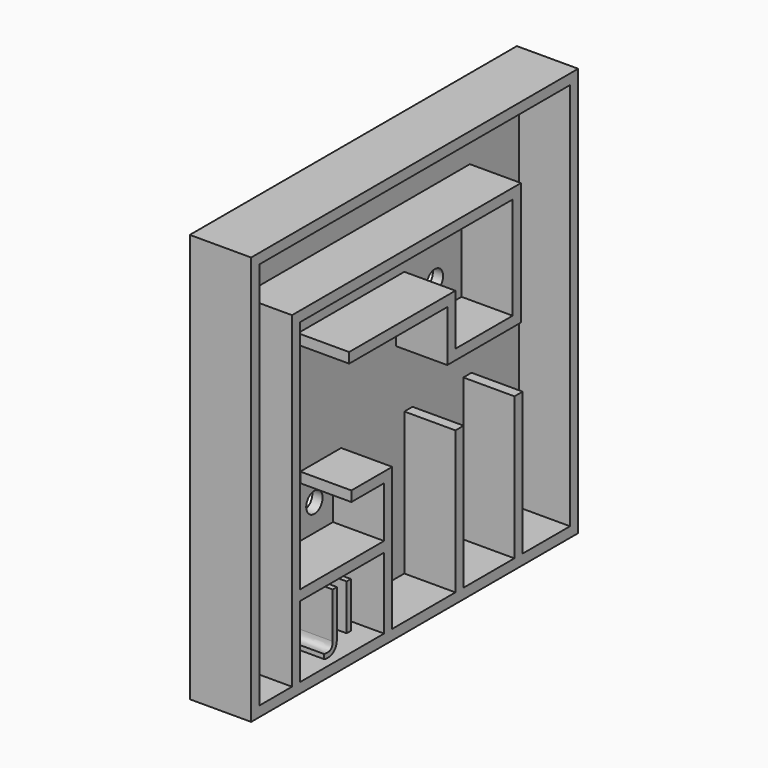
from build123d import *

# Parameters (mm, degrees)
F0_W          = 50.8
F0_H          = 50.8
F1_DEPTH      = 7.62
F2_T          = -1.27
F3_W          = 1.27
F3_H          = 40.64
F4_DEPTH      = 6.35
F5_R          = 1.27
F6_DEPTH      = 2540
F7_DEPTH      = 25.4
F10_DEPTH     = 6.35
F8_W          = 34.29
F8_H          = 1.27
F11_DEPTH     = 6.35
F12_W         = 1.27
F12_H         = 1.27
F12_W_2       = 15.24
F12_W_3       = 5.08
F12_W_4       = 13.0282191968
F12_H_2       = 17.7213940769
F13_DEPTH     = 6.35
F14_TEXT_SIZE = 7.9484365415
F15_DEPTH     = 6.35
F16_R         = 1.27
F17_DEPTH     = 254


# Not quite as in the source:
# - Text() gives the source's letters only with a copy of the font that has no kerning and outlines rounded to 1/6400 em; it was checked with that copy


with BuildPart() as f1:
    # F0 (on Right) → F1 (new body)
    with BuildSketch(Plane.YZ):
        with Locations((-25.4, 25.4)):
            Rectangle(F0_W, F0_H)
    extrude(amount=F1_DEPTH)

    # F2
    f2_openings = [f1.faces().sort_by_distance(p)[0] for p in [
        (7.62, -25.4, 25.4),
    ]]
    offset(amount=F2_T, openings=f2_openings)

    # F3 (on face) → F4 (join)
    with BuildSketch(Plane.YZ.offset(1.27)):
        with Locations((-43.815, 21.59)):
            Rectangle(F3_W, F3_H)
    extrude(amount=F4_DEPTH)

    # F5 (on face) → F6 (cut)
    with BuildSketch(Plane.YZ.offset(1.27)):
        with Locations((-46.99, 3.81)):
            Circle(F5_R)
        with Locations((-46.99, 11.43)):
            Circle(F5_R)
    extrude(amount=-F6_DEPTH, mode=Mode.SUBTRACT)

    # F5 (on face) → F7 (cut)
    with BuildSketch(Plane.YZ.offset(1.27)):
        with Locations((-46.99, 3.81)):
            Circle(F5_R)
        with Locations((-46.99, 11.43)):
            Circle(F5_R)
        with Locations((-46.99, 20.32)):
            Circle(F5_R)
    extrude(amount=-F7_DEPTH, mode=Mode.SUBTRACT)

    # F9 (on face) → F10 (join)
    with BuildSketch(Plane.YZ.offset(1.27)):
        Polygon((-8.9077808741, 26.6518555582), (-8.9077808741, 39.3518555582), (-8.9077808741, 40.6393446028), (-10.1777808741, 40.876660496), (-10.1777808741, 27.9218555582), (-19.0677808741, 27.9218555582), (-19.0677808741, 26.6518555582), align=None)
    extrude(amount=F10_DEPTH)

    # F8 (on face) → F11 (join)
    with BuildSketch(Plane.YZ.offset(1.27)):
        with Locations((-26.035, 41.275)):
            Rectangle(F8_W, F8_H)
    extrude(amount=F11_DEPTH)

    # F12 (on face) → F13 (join)
    with BuildSketch(Plane.YZ.offset(1.27)):
        with Locations((-19.7027808741, 33.6368555582)):
            Rectangle(F12_W, F12_H)
        with Locations((-27.9577808741, 33.6368555582)):
            Rectangle(F12_W_2, F12_H)
        with Locations((-32.6917808032, 18.3563940769)):
            Rectangle(F12_W_3, F12_H)
        Polygon((-30.1517808032, 16.935095191), (-30.1517808032, 11.4006970385), (-30.1517808032, 10.1306970385), (-30.1517808032, 1.27), (-28.8817808032, 1.27), (-28.8817808032, 18.9913940769), (-30.1517808032, 18.9913940769), (-30.1517808032, 17.7213940769), align=None)
        with Locations((-36.6658904016, 10.7656970385)):
            Rectangle(F12_W_4, F12_H)
        with Locations((-18.4327808741, 10.1306970385)):
            Rectangle(F12_W, F12_H_2)
        with Locations((-9.2695793679, 10.1306970385)):
            Rectangle(F12_W, F12_H_2)
        Polygon((-19.0677808741, 26.6518555582), (-19.0677808741, 27.9218555582), (-19.0677808741, 33.0018555582), (-20.3377808741, 33.0018555582), (-20.3377808741, 31.5799154341), (-20.3377808741, 26.6518555582), align=None)
    extrude(amount=F13_DEPTH)

    # F14 (on face) → F15 (join)
    with BuildSketch(Plane.YZ.offset(1.27)):
        with Locations((-38.8736948371, 3.6668670364)):
            Text('JI', F14_TEXT_SIZE, font='Open Sans', text_align=(TextAlign.LEFT, TextAlign.BOTTOM))
    extrude(amount=F15_DEPTH)

    # F16 (on face) → F17 (cut)
    with BuildSketch(Plane.YZ.offset(1.27)):
        with Locations((-14.3160289153, 31.3759669662)):
            Circle(F16_R)
        with Locations((-33.0355912447, 14.7394770756)):
            Circle(F16_R)
        with Locations((-13.4074687958, 4.6649156138)):
            Circle(F16_R)
    extrude(amount=-F17_DEPTH, mode=Mode.SUBTRACT)


solid = f1.part
